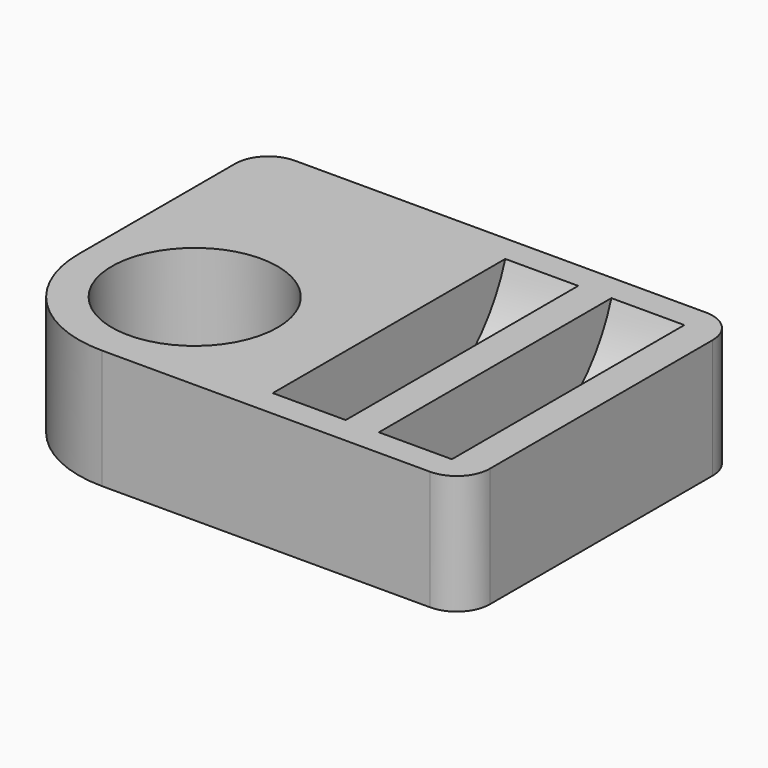
from build123d import *

# Parameters (mm, degrees)
F0_R         = 12.5
F1_DEPTH     = 25
F2_W         = 11
F2_H         = 23
F4_W         = 82.2123259306
F4_H         = 18.054354161
F5_DEPTH     = 52.001
F6_TEXT_SIZE = 5.5555555556
F7_DEPTH     = 1


# Not quite as in the source:
# - Text() gives the source's letters only with a copy of the font that has no kerning and outlines rounded to 1/6400 em; it was checked with that copy


with BuildPart() as f1:
    # F0 (on Top) → F1 (new body)
    with BuildSketch(Plane.XY):
        with BuildLine():
            ThreePointArc((0, 17.5), (5.1256313292, 5.1256313292), (17.5, 0))
            Line((17.5, 0), (67, 0))
            ThreePointArc((67, 0), (70.5355339059, 1.4644660941), (72, 5))
            Line((72, 5), (72, 47))
            ThreePointArc((72, 47), (70.5355339059, 50.5355339059), (67, 52))
            Line((67, 52), (5, 52))
            ThreePointArc((5, 52), (1.4644660941, 50.5355339059), (0, 47))
            Line((0, 47), (0, 17.5))
        make_face()
        with Locations((17.5, 17.5)):
            Circle(F0_R, mode=Mode.SUBTRACT)
    extrude(amount=F1_DEPTH)

    # F2 (on face) → F3 (revolve, cut)
    with BuildSketch(Plane.XY.offset(25)):
        with Locations((45.5, 14.5)):
            Rectangle(F2_W, F2_H)
        with Locations((61.5, 14.5)):
            Rectangle(F2_W, F2_H)
    revolve(axis=Axis((45.5, 26, 25), (1, 0, 0)), mode=Mode.SUBTRACT)

    # F4 (on face) → F5 (cut, through all)
    with BuildSketch(Plane.XZ):
        with Locations((41.1061629653, 27.0271770805)):
            Rectangle(F4_W, F4_H)
    extrude(amount=-F5_DEPTH, mode=Mode.SUBTRACT)

    # F6 (on face) → F7 (cut)
    with BuildSketch(Plane(origin=(0, 0, 0), x_dir=(1, 0, 0), z_dir=(0, 0, -1))):
        with Locations((30, -9)):
            Text('841', F6_TEXT_SIZE, font='Open Sans', text_align=(TextAlign.LEFT, TextAlign.BOTTOM))
    extrude(amount=-F7_DEPTH, mode=Mode.SUBTRACT)


solid = f1.part
